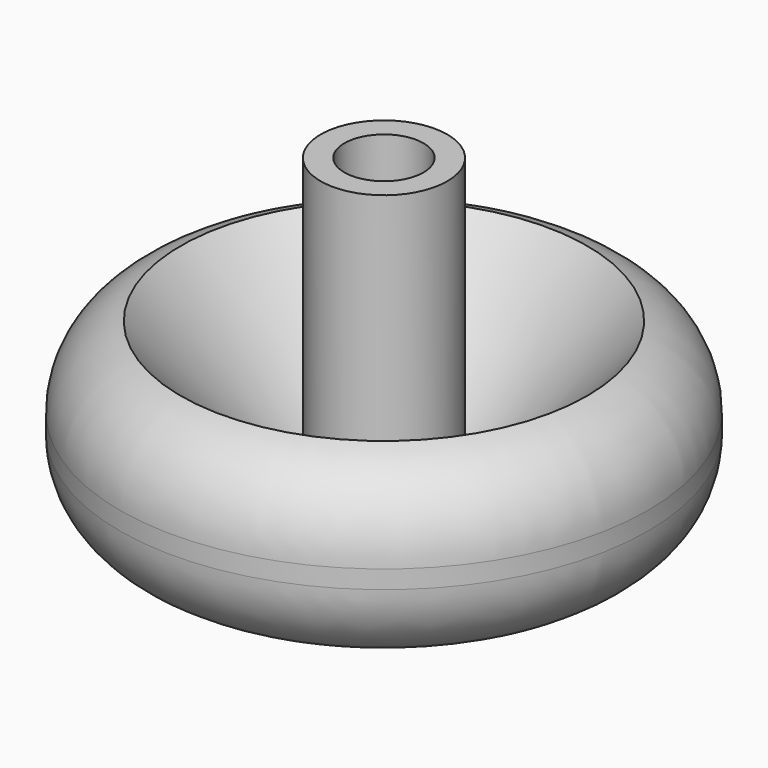
from build123d import *

# Parameters (mm, degrees)
F3_R     = 25.4
F4_R     = 4.7625
F5_DEPTH = 9.525
F6_R     = 1.5875
F7_DEPTH = 9.525


# Not quite as in the source:
# - a fillet or chamfer that OpenCascade refuses, or shapes differently, is made with other operations: its cross-section is extruded or revolved along the edge and cut away or added


with BuildPart() as f1:
    # F0 (on Front) → F1 (revolve)
    with BuildSketch(Plane.XZ):
        Polygon((10.5000606809, 4.0159458295), (31.75, 8.134865202), (31.75, 28.454865202), (24.4433090497, 28.454865202), (7.62, 9.4384327507), (7.62, 45.72), (0, 45.72), (0, 0), (1.5875, 0), align=None)
    revolve(axis=Axis((0, 0, 22.86), (0, 0, -1)))

    # F2: fillet of radius 10.16 on 3 edges, made by hand

    # F2_s1 → F2_t2 (revolve, cut)
    with BuildSketch(Plane.XZ):
        with BuildLine():
            ThreePointArc((23.5233497224, 6.5402766862), (29.4279982514, 10.0500062027), (31.75, 16.5146317456))
            Line((31.75, 16.5146317456), (31.75, 8.134865202))
            Line((31.75, 8.134865202), (23.5233497224, 6.5402766862))
        make_face()
    revolve(axis=Axis((0, 0, 8.134865202), (0, 0, -1)), mode=Mode.SUBTRACT)

    # F2_s3 → F2_t4 (revolve, cut)
    with BuildSketch(Plane.XZ):
        with BuildLine():
            ThreePointArc((31.75, 18.7037510366), (29.7206586432, 24.7962045676), (24.4433090497, 28.454865202))
            Line((24.4433090497, 28.454865202), (31.75, 28.454865202))
            Line((31.75, 28.454865202), (31.75, 18.7037510366))
        make_face()
    revolve(axis=Axis((0, 0, 28.454865202), (0, 0, -1)), mode=Mode.SUBTRACT)

    # F3
    f3_edges = [f1.edges().sort_by_distance(p)[0] for p in [
        (-10.500061, 0, 4.015946),
    ]]
    fillet(f3_edges, radius=F3_R)

    # F4 (on face) → F5 (cut)
    with BuildSketch(Plane.XY.offset(45.72)):
        Circle(F4_R)
    extrude(amount=-F5_DEPTH, mode=Mode.SUBTRACT)

    # F6 (on Top) → F7 (cut)
    with BuildSketch(Plane.XY):
        Circle(F6_R)
    extrude(amount=F7_DEPTH, mode=Mode.SUBTRACT)


solid = f1.part
